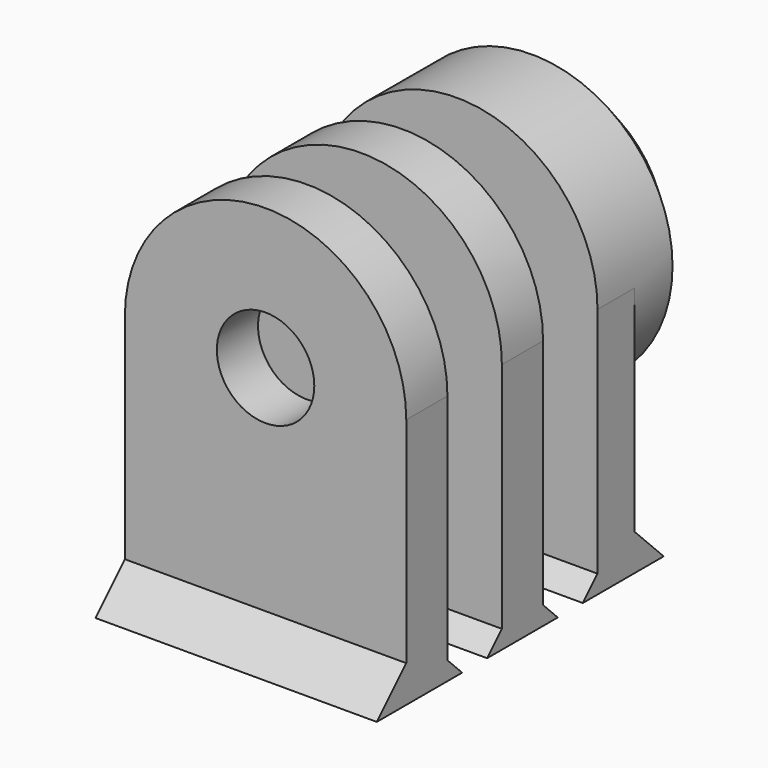
from build123d import *

# Parameters (mm, degrees)
F0_R      = 2.65
F1_DEPTH  = 1.4
F2_START  = 5.1
F2_DEPTH  = 2.8
F3_START  = -5.1
F3_DEPTH  = 2.5
F4_START  = -7.5
F4_DEPTH  = 4.7
F5_SIZE   = 2
F10_DEPTH = 15.3


# Not quite as in the source:
# - a feature names something its author has since deleted; it is built from what else it names


with BuildPart() as f1:
    # F0 (on Front) → F1 (new body, symmetric)
    with BuildSketch(Plane.XZ):
        with BuildLine():
            ThreePointArc((-7.65, 0), (0, -7.65), (7.65, 0))
            ThreePointArc((7.65, 0), (0, 7.65), (-7.65, 0))
        make_face()
        Polygon((2.3094010768, 4), (4.6188021535, 0), (2.3094010768, -4), (-2.3094010768, -4), (-4.6188021535, 0), (-2.3094010768, 4), align=None, mode=Mode.SUBTRACT)
        Polygon((2.3094010768, -4), (4.6188021535, 0), (2.3094010768, 4), (-2.3094010768, 4), (-4.6188021535, 0), (-2.3094010768, -4), align=None)
        Circle(F0_R, mode=Mode.SUBTRACT)
        with BuildLine():
            Line((7.65, -13.65), (7.65, 0))
            ThreePointArc((7.65, 0), (0, -7.65), (-7.65, 0))
            Line((-7.65, 0), (-7.65, -13.65))
            Line((-7.65, -13.65), (7.65, -13.65))
        make_face()
    extrude(amount=F1_DEPTH, both=True)

    # F9 (on face) → F10, piece 2 (join, through all)
    with BuildSketch(Plane(origin=(-7.65, 0, 0), x_dir=(0, -1, 0), z_dir=(-1, 0, 0))):
        Polygon((-2.4, -13.65), (-1.4, -13.65), (-1.4, -12.65), align=None)
        Polygon((1.4, -12.65), (1.4, -13.65), (2.4, -13.65), align=None)
    extrude(amount=-F10_DEPTH)


with BuildPart() as f2:
    # F0 (on Front) → F2 (new body)
    with BuildSketch(Plane.XZ.offset(F2_START)):
        with BuildLine():
            ThreePointArc((-7.65, 0), (0, -7.65), (7.65, 0))
            ThreePointArc((7.65, 0), (0, 7.65), (-7.65, 0))
        make_face()
        Polygon((2.3094010768, 4), (4.6188021535, 0), (2.3094010768, -4), (-2.3094010768, -4), (-4.6188021535, 0), (-2.3094010768, 4), align=None, mode=Mode.SUBTRACT)
        Polygon((2.3094010768, -4), (4.6188021535, 0), (2.3094010768, 4), (-2.3094010768, 4), (-4.6188021535, 0), (-2.3094010768, -4), align=None)
        Circle(F0_R, mode=Mode.SUBTRACT)
        with BuildLine():
            Line((7.65, -13.65), (7.65, 0))
            ThreePointArc((7.65, 0), (0, -7.65), (-7.65, 0))
            Line((-7.65, 0), (-7.65, -13.65))
            Line((-7.65, -13.65), (7.65, -13.65))
        make_face()
    extrude(amount=F2_DEPTH)

    # F7 (on face) + F9 (on face) → F10, piece 3 (join, through all)
    with BuildSketch(Plane(origin=(-7.65, 0, 0), x_dir=(0, -1, 0), z_dir=(-1, 0, 0))):
        Polygon((7.9, -11.65), (7.9, -13.65), (9.9, -13.65), align=None)
    with BuildSketch(Plane(origin=(-7.65, 0, 0), x_dir=(0, -1, 0), z_dir=(-1, 0, 0))):
        Polygon((4.1, -13.65), (5.1, -13.65), (5.1, -12.65), align=None)
    extrude(amount=-F10_DEPTH)


with BuildPart() as f3:
    # F0 (on Front) → F3 (new body)
    with BuildSketch(Plane.XZ.offset(F3_START)):
        with BuildLine():
            ThreePointArc((-7.65, 0), (0, -7.65), (7.65, 0))
            ThreePointArc((7.65, 0), (0, 7.65), (-7.65, 0))
        make_face()
        Polygon((2.3094010768, 4), (4.6188021535, 0), (2.3094010768, -4), (-2.3094010768, -4), (-4.6188021535, 0), (-2.3094010768, 4), align=None, mode=Mode.SUBTRACT)
        Polygon((2.3094010768, -4), (4.6188021535, 0), (2.3094010768, 4), (-2.3094010768, 4), (-4.6188021535, 0), (-2.3094010768, -4), align=None)
        Circle(F0_R, mode=Mode.SUBTRACT)
        with BuildLine():
            Line((7.65, -13.65), (7.65, 0))
            ThreePointArc((7.65, 0), (0, -7.65), (-7.65, 0))
            Line((-7.65, 0), (-7.65, -13.65))
            Line((-7.65, -13.65), (7.65, -13.65))
        make_face()
    extrude(amount=-F3_DEPTH)

    # F0 (on Front) → F4 (join)
    with BuildSketch(Plane.XZ.offset(F4_START)):
        with BuildLine():
            ThreePointArc((-7.65, 0), (0, -7.65), (7.65, 0))
            ThreePointArc((7.65, 0), (0, 7.65), (-7.65, 0))
        make_face()
        Polygon((2.3094010768, 4), (4.6188021535, 0), (2.3094010768, -4), (-2.3094010768, -4), (-4.6188021535, 0), (-2.3094010768, 4), align=None, mode=Mode.SUBTRACT)
    extrude(amount=-F4_DEPTH)

    # F5
    f5_edges = [f3.edges().sort_by_distance(p)[0] for p in [
        (-7.65, 12.2, 0),
    ]]
    chamfer(f5_edges, length=F5_SIZE)

    # F6 (on face) + F8 (on face) → F10 (join, through all)
    with BuildSketch(Plane(origin=(-7.65, 0, 0), x_dir=(0, -1, 0), z_dir=(-1, 0, 0))):
        Polygon((-9.6, -13.65), (-7.6, -13.65), (-7.6, -11.65), align=None)
    with BuildSketch(Plane(origin=(-7.65, 0, 0), x_dir=(0, -1, 0), z_dir=(-1, 0, 0))):
        Polygon((-5.1, -12.65), (-5.1, -13.65), (-4.1, -13.65), align=None)
    extrude(amount=-F10_DEPTH)


solid = Compound([f1.part, f2.part, f3.part])
